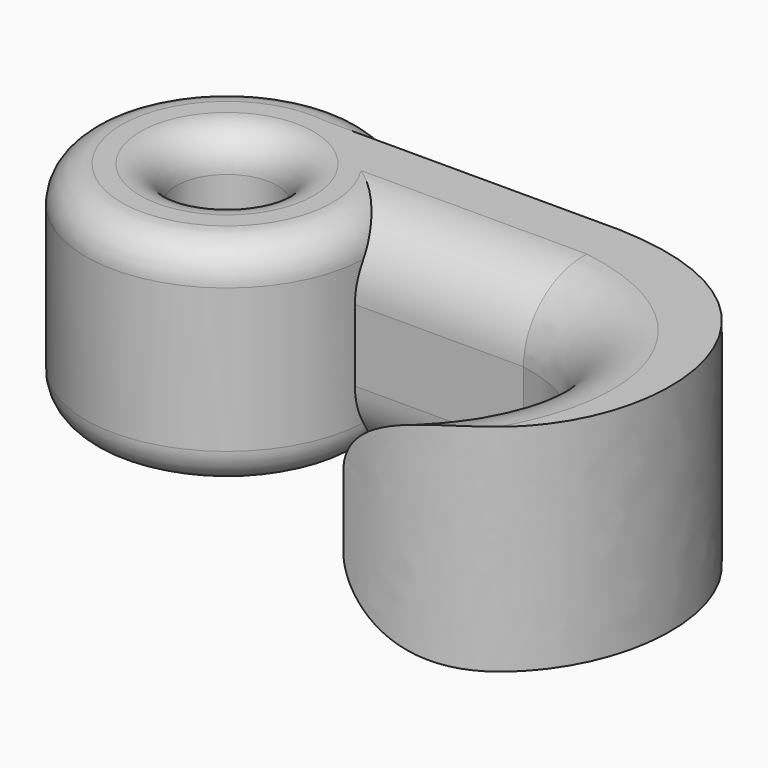
from build123d import *

# Parameters (mm, degrees)
F0_R     = 1.7947651686
F1_DEPTH = 7.62
F2_R     = 2.54
F3_R     = 1.269


# Not quite as in the source:
# - a fillet or chamfer is up to 0.001 mm smaller than in the source, because OpenCascade refuses the exact size


with BuildPart() as f1:
    # F0 (on Top) → F1 (new body)
    with BuildSketch(Plane.XY):
        with BuildLine():
            ThreePointArc((-3.0625740785, 3.6819641418), (-1.865183548, 2.011379827), (-1.4421620036, 0))
            ThreePointArc((-1.4421620036, 0), (-1.4498583422, -0.2771315824), (-1.4729236329, -0.5534088705))
            Line((-1.4729236329, -0.5534088705), (4.4801407494, -0.5534088705))
            Line((4.4801407494, -0.5534088705), (4.4801407494, 3.6819641418))
            Line((4.4801407494, 3.6819641418), (-3.0625740785, 3.6819641418))
        make_face()
        with BuildLine():
            add(Edge.make_bspline(
                [(4.4801407494, 3.6819641418), (14.6919268718, 3.3504103776), (12.7431834117, -10.4070426896), (4.4801407494, -8.5037574172)],
                knots=[0, 0, 0, 0, 12.185721559, 12.185721559, 12.185721559, 12.185721559], degree=3))
            Line((4.4801407494, 3.6819641418), (4.4801407494, -0.5534088705))
            add(Edge.make_bspline(
                [(4.4801407494, -0.5534088705), (9.772202, -1.5405191807), (7.8137687942, -7.3264148086), (4.4801407494, -8.5037574172)],
                knots=[0, 0, 0, 0, 7.9503485467, 7.9503485467, 7.9503485467, 7.9503485467], degree=3))
        make_face()
        with BuildLine():
            ThreePointArc((-1.4729236329, -0.5534088705), (-1.4498583422, -0.2771315824), (-1.4421620036, 0))
            ThreePointArc((-1.4421620036, 0), (-1.865183548, 2.011379827), (-3.0625740785, 3.6819641418))
            ThreePointArc((-3.0625740785, 3.6819641418), (-11.1104438204, -1.7546257881), (-1.4729236329, -0.5534088705))
        make_face()
        with Locations((-6.4355200157, 0)):
            Circle(F0_R, mode=Mode.SUBTRACT)
    extrude(amount=F1_DEPTH)

    # F2
    f2_edges = [f1.edges().sort_by_distance(p)[0] for p in [
        (1.503609, -0.553409, 7.62),
        (7.731849, -4.321745, 7.62),
        (1.503609, -0.553409, 0),
        (7.731849, -4.321745, 0),
    ]]
    fillet(f2_edges, radius=F2_R)

    # F3 (radius 1.27 in the source; OpenCascade refuses exactly that, so slightly less here)
    f3_edges = [f1.edges().sort_by_distance(p)[0] for p in [
        (-11.110444, -1.754626, 7.62),
        (-11.110444, -1.754626, 0),
        (-8.230285, 0, 0),
        (-8.230285, 0, 7.62),
    ]]
    fillet(f3_edges, radius=F3_R)


solid = f1.part
